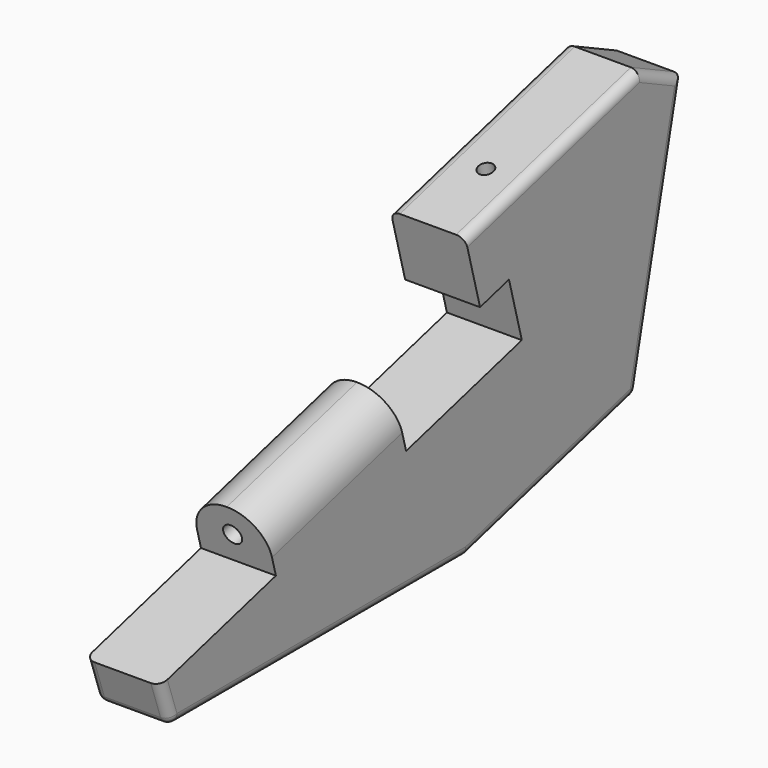
from build123d import *

# Parameters (mm, degrees)
F1_DEPTH = 20
F3_D     = 10
F3_DEPTH = 90
F3_TIP   = 3.0043030951
F4_R     = 19.99999
F5_R     = 5
F7_D     = 8


# Not quite as in the source:
# - a fillet or chamfer is up to 0.001 mm smaller than in the source, because OpenCascade refuses the exact size


with BuildPart() as f1:
    # F0 (on Right) → F1 (new body, symmetric)
    with BuildSketch(Plane.YZ):
        Polygon((55.3865908633, 32.2499277236), (-31.5467335027, 8.9562136644), (-23.7821621496, -20.0215611243), (-101.0562282528, -40.7270847325), (-93.3750867844, -62.9337131977), (103.556553434, -62.9337131977), (217.0635979758, -32.5195922775), (248.1942623854, 104.8115119338), (219.449320977, 118.5184651202), (102.765125102, 87.253029066), (112.5305330656, 50.8080303895), (131.8490495913, 55.9844112915), (140.4252283195, 23.9776765432), (63.1511622164, 3.272152935), align=None)
    extrude(amount=F1_DEPTH, both=True)

    # F3
    with Locations(Plane(origin=(0, -27.1944496451, -7.286730821), x_dir=(1, 0, 0), z_dir=(0, -0.9659258263, -0.2588190451))):
        with Locations((0, 1.8159335255)):
            Hole(F3_D / 2, depth=F3_DEPTH)
            with Locations((0, 0, -(F3_DEPTH + F3_TIP / 2))):  # 118° drill point
                Cone(0, F3_D / 2, F3_TIP, mode=Mode.SUBTRACT)

    # F4 (radius 20 in the source; OpenCascade refuses exactly that, so slightly less here)
    f4_edges = [f1.edges().sort_by_distance(p)[0] for p in [
        (20, 11.919929, 20.603071),
        (-20, 11.919929, 20.603071),
    ]]
    fillet(f4_edges, radius=F4_R)

    # F5
    f5_edges = [f1.edges().sort_by_distance(p)[0] for p in [
        (-20, -97.215658, -51.830399),
        (20, -97.215658, -51.830399),
        (0, -93.375087, -62.933713),
        (20, 5.090733, -62.933713),
        (-20, 5.090733, -62.933713),
        (20, 160.310076, -47.726653),
        (-20, 160.310076, -47.726653),
        (0, 217.063598, -32.519592),
        (20, 232.62893, 36.14596),
        (-20, 232.62893, 36.14596),
        (-20, 233.821792, 111.664989),
        (20, 233.821792, 111.664989),
        (20, 161.107223, 102.885747),
        (-20, 161.107223, 102.885747),
    ]]
    fillet(f5_edges, radius=F5_R)

    # F7 (through all)
    with Locations(Plane(origin=(0, -14.9292991962, 55.7169031216), x_dir=(1, 0, 0), z_dir=(0, -0.2588190451, 0.9659258263))):
        with Locations((0, 161.846234043)):
            Hole(F7_D / 2)


solid = f1.part
